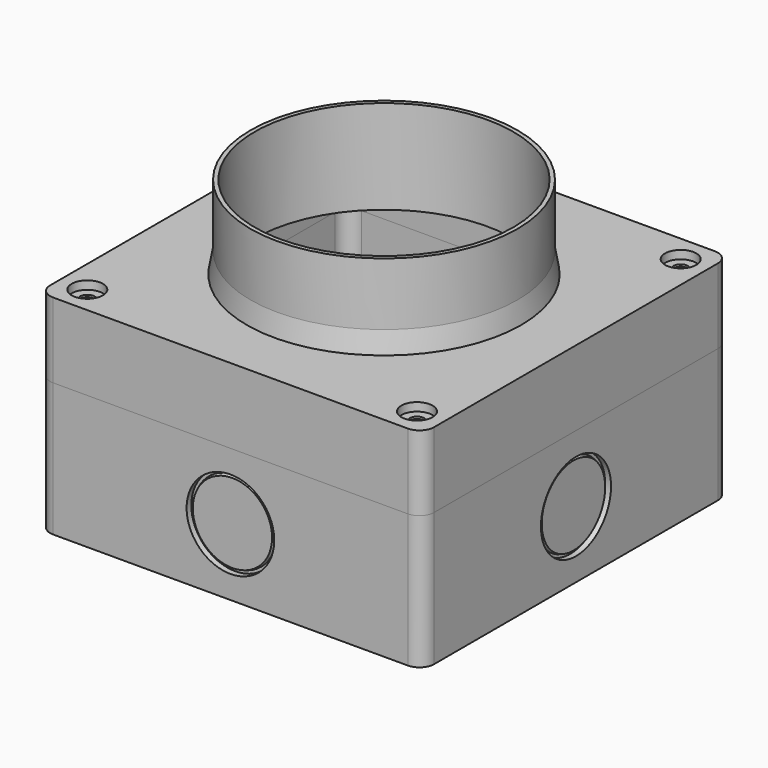
from build123d import *

# Parameters (mm, degrees)
F0_W      = 92
F0_H      = 92
F1_DEPTH  = 3
F4_W      = 92
F4_H      = 92
F4_W_2    = 89
F4_H_2    = 89
F5_DEPTH  = 29
F6_R      = 3.5
F7_R      = 10.5
F8_DEPTH  = 1.4
F9_R      = 10
F10_DEPTH = 0.8
F12_R     = 10.5
F13_DEPTH = 1.4
F14_R     = 10
F15_DEPTH = 0.8
F17_R     = 10.5
F18_DEPTH = 1.4
F19_R     = 10
F20_DEPTH = 0.8
F22_R     = 10.5
F23_DEPTH = 1.4
F24_R     = 10
F25_DEPTH = 0.8
F28_W     = 92
F28_H     = 92
F28_W_2   = 89
F28_H_2   = 89
F29_DEPTH = 15.5
F30_W     = 92
F30_H     = 92
F31_DEPTH = 2.5
F32_R     = 3.5
F33_R     = 3.75
F34_DEPTH = 2
F35_R     = 1.75
F36_DEPTH = 2.5
F37_R     = 1.75
F38_DEPTH = 2.5
F39_R     = 1.75
F40_DEPTH = 25
F41_R     = 1.75
F42_DEPTH = 25
F43_R     = 33
F44_DEPTH = 5
F46_R     = 32
F47_DEPTH = 15
F48_R     = 31
F49_DEPTH = 25


# Not quite as in the source:
# - a fillet or chamfer that OpenCascade refuses, or shapes differently, is made with other operations: its cross-section is extruded or revolved along the edge and cut away or added
# - a feature of the source that left no trace in its solid (it failed there, or was rolled back) is left out


with BuildPart() as f1:
    # F0 (on Top) → F1 (new body)
    with BuildSketch(Plane.XY):
        Rectangle(F0_W, F0_H)
    extrude(amount=F1_DEPTH)

    # F4 (on offset) → F5 (join)
    with BuildSketch(Plane.XY.offset(3)):
        Rectangle(F4_W, F4_H)
        Rectangle(F4_W_2, F4_H_2, mode=Mode.SUBTRACT)
    extrude(amount=F5_DEPTH)

    # F6
    f6_edges = [f1.edges().sort_by_distance(p)[0] for p in [
        (-44.5, -44.5, 17.5),
        (-46, -46, 16),
        (-46, 46, 16),
        (-44.5, 44.5, 17.5),
        (46, 46, 16),
        (44.5, 44.5, 17.5),
        (46, -46, 16),
        (44.5, -44.5, 17.5),
    ]]
    fillet(f6_edges, radius=F6_R)

    # F7 (on face) → F8 (cut)
    with BuildSketch(Plane.XZ.offset(46)):
        with Locations((0, 16)):
            Circle(F7_R)
    extrude(amount=-F8_DEPTH, mode=Mode.SUBTRACT)

    # F9 (on face) → F10 (join)
    with BuildSketch(Plane.XZ.offset(44.6)):
        with Locations((0, 16)):
            Circle(F9_R)
    extrude(amount=F10_DEPTH)

    # F11: chamfer of 0.5 x 1.3737387097 on 1 edges, made by hand


with BuildPart() as f11_tool2:
    # F11_s3 → F11_t4 (revolve)
    with BuildSketch(Plane.XY.offset(16)):
        Polygon((10, -44.0262612903), (9.5, -45.4), (10, -45.4), align=None)
    revolve(axis=Axis((0, -45.4, 16), (0, -1, 0)))

    split(bisect_by=Plane.XZ.offset(44.6), keep=Keep.TOP)


with BuildPart() as f1_1:
    add(f1.part)

    # F11_t1: cut F11_tool2
    add(f11_tool2.part, mode=Mode.SUBTRACT)

    # F12 (on face) → F13 (cut)
    with BuildSketch(Plane(origin=(-46, 0, 0), x_dir=(0, -1, 0), z_dir=(-1, 0, 0))):
        with Locations((0, 16)):
            Circle(F12_R)
    extrude(amount=-F13_DEPTH, mode=Mode.SUBTRACT)

    # F14 (on face) → F15 (join)
    with BuildSketch(Plane(origin=(-44.6, 0, 0), x_dir=(0, -1, 0), z_dir=(-1, 0, 0))):
        with Locations((0, 16)):
            Circle(F14_R)
    extrude(amount=F15_DEPTH)

    # F16: chamfer of 0.5 x 1.3737387097 on 1 edges, made by hand


with BuildPart() as f16_tool2:
    # F16_s3 → F16_t4 (revolve)
    with BuildSketch(Plane.XY.offset(16)):
        Polygon((-44.0262612903, -10), (-45.4, -9.5), (-45.4, -10), align=None)
    revolve(axis=Axis((-45.4, 0, 16), (-1, 0, 0)))

    split(bisect_by=Plane.YZ.offset(-44.6), keep=Keep.BOTTOM)


with BuildPart() as f1_2:
    add(f1_1.part)

    # F16_t1: cut F16_tool2
    add(f16_tool2.part, mode=Mode.SUBTRACT)

    # F17 (on face) → F18 (cut)
    with BuildSketch(Plane(origin=(0, 46, 0), x_dir=(-1, 0, 0), z_dir=(0, 1, 0))):
        with Locations((0, 16)):
            Circle(F17_R)
    extrude(amount=-F18_DEPTH, mode=Mode.SUBTRACT)

    # F19 (on face) → F20 (join)
    with BuildSketch(Plane(origin=(0, 44.6, 0), x_dir=(-1, 0, 0), z_dir=(0, 1, 0))):
        with Locations((0, 16)):
            Circle(F19_R)
    extrude(amount=F20_DEPTH)

    # F21: chamfer of 0.5 x 1.3737387097 on 1 edges, made by hand


with BuildPart() as f21_tool2:
    # F21_s3 → F21_t4 (revolve)
    with BuildSketch(Plane.XY.offset(16)):
        Polygon((-10, 44.0262612903), (-9.5, 45.4), (-10, 45.4), align=None)
    revolve(axis=Axis((0, 45.4, 16), (0, 1, 0)))

    split(bisect_by=Plane.XZ.offset(-44.6), keep=Keep.BOTTOM)


with BuildPart() as f1_3:
    add(f1_2.part)

    # F21_t1: cut F21_tool2
    add(f21_tool2.part, mode=Mode.SUBTRACT)

    # F22 (on face) → F23 (cut)
    with BuildSketch(Plane.YZ.offset(46)):
        with Locations((0, 16)):
            Circle(F22_R)
    extrude(amount=-F23_DEPTH, mode=Mode.SUBTRACT)

    # F24 (on face) → F25 (join)
    with BuildSketch(Plane.YZ.offset(44.6)):
        with Locations((0, 16)):
            Circle(F24_R)
    extrude(amount=F25_DEPTH)

    # F26: chamfer of 0.5 x 1.3737387097 on 1 edges, made by hand


with BuildPart() as f26_tool2:
    # F26_s3 → F26_t4 (revolve)
    with BuildSketch(Plane.XY.offset(16)):
        Polygon((44.0262612903, 10), (45.4, 9.5), (45.4, 10), align=None)
    revolve(axis=Axis((45.4, 0, 16), (1, 0, 0)))

    split(bisect_by=Plane.YZ.offset(44.6), keep=Keep.TOP)


with BuildPart() as f1_4:
    add(f1_3.part)

    # F26_t1: cut F26_tool2
    add(f26_tool2.part, mode=Mode.SUBTRACT)


with BuildPart() as f29:
    # F28 (on offset) → F29 (new body)
    with BuildSketch(Plane.XY.offset(32)):
        Rectangle(F28_W, F28_H)
        Rectangle(F28_W_2, F28_H_2, mode=Mode.SUBTRACT)
    extrude(amount=F29_DEPTH)

    # F30 (on face) → F31 (join)
    with BuildSketch(Plane.XY.offset(47.5)):
        Rectangle(F30_W, F30_H)
    extrude(amount=F31_DEPTH)

    # F32
    f32_edges = [f29.edges().sort_by_distance(p)[0] for p in [
        (-46, -46, 41),
        (-44.5, -44.5, 39.75),
        (46, -46, 41),
        (44.5, -44.5, 39.75),
        (44.5, 44.5, 39.75),
        (46, 46, 41),
        (-46, 46, 41),
        (-44.5, 44.5, 39.75),
    ]]
    fillet(f32_edges, radius=F32_R)

    # F33 (on face) → F34 (cut)
    with BuildSketch(Plane.XY.offset(50)):
        with Locations((-39.5, 39.5)):
            Circle(F33_R)
        with Locations((39.5, 39.5)):
            Circle(F33_R)
        with Locations((39.5, -39.5)):
            Circle(F33_R)
        with Locations((-39.5, -39.5)):
            Circle(F33_R)
    extrude(amount=-F34_DEPTH, mode=Mode.SUBTRACT)

    # F35 (on face) → F36 (cut)
    with BuildSketch(Plane.XY.offset(48)):
        with Locations((-39.5, 39.5)):
            Circle(F35_R)
    extrude(amount=-F36_DEPTH, mode=Mode.SUBTRACT)

    # F37 (on face) → F38 (cut)
    with BuildSketch(Plane.XY.offset(48)):
        with Locations((39.5, 39.5)):
            Circle(F37_R)
    extrude(amount=-F38_DEPTH, mode=Mode.SUBTRACT)

    # F39 (on face) → F40 (cut)
    with BuildSketch(Plane.XY.offset(48)):
        with Locations((39.5, -39.5)):
            Circle(F39_R)
    extrude(amount=-F40_DEPTH, mode=Mode.SUBTRACT)

    # F41 (on face) → F42 (cut)
    with BuildSketch(Plane.XY.offset(48)):
        with Locations((-39.5, -39.5)):
            Circle(F41_R)
    extrude(amount=-F42_DEPTH, mode=Mode.SUBTRACT)

    # F43 (on face) → F44 (join)
    with BuildSketch(Plane.XY.offset(50)):
        Circle(F43_R)
    extrude(amount=F44_DEPTH)

    # F45: chamfer of 1 x 5.6712818196 on 1 edges, made by hand


with BuildPart() as f45_tool2:
    # F45_s3 → F45_t4 (revolve)
    with BuildSketch(Plane.XZ):
        Polygon((33, 49.3287181804), (32, 55), (33, 55), align=None)
    revolve(axis=Axis((0, 0, 55), (0, 0, 1)))

    split(bisect_by=Plane.XY.offset(50), keep=Keep.TOP)


with BuildPart() as f29_1:
    add(f29.part)

    # F45_t1: cut F45_tool2
    add(f45_tool2.part, mode=Mode.SUBTRACT)

    # F46 (on face) → F47 (join)
    with BuildSketch(Plane.XY.offset(55)):
        Circle(F46_R)
    extrude(amount=F47_DEPTH)

    # F48 (on face) → F49 (cut)
    with BuildSketch(Plane.XY.offset(70)):
        Circle(F48_R)
    extrude(amount=-F49_DEPTH, mode=Mode.SUBTRACT)


solid = Compound([f1_4.part, f29_1.part])
